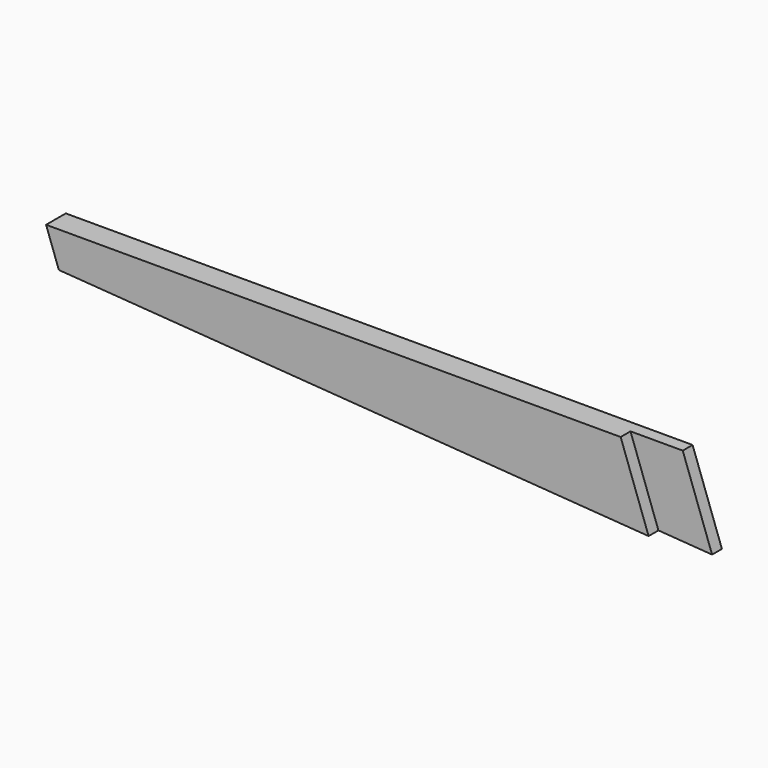
from build123d import *

# Parameters (mm, degrees)
F0_W     = 508
F0_H     = 63.5
F1_DEPTH = 19.05
F3_DEPTH = 50.8
F5_DEPTH = 50.8
F7_DEPTH = 38.1
F9_DEPTH = 38.1


with BuildPart() as f1:
    # F0 (on Front) → F1 (new body)
    with BuildSketch(Plane.XZ):
        with Locations((7.0352284261, 31.75)):
            Rectangle(F0_W, F0_H)
    extrude(amount=F1_DEPTH)

    # F2 (on face) → F3 (cut)
    with BuildSketch(Plane.XZ.offset(19.05)):
        Polygon((-224.2599035735, 0), (-246.9647715739, 63.5), (-246.9647715739, 0), align=None)
    extrude(amount=-F3_DEPTH, mode=Mode.SUBTRACT)

    # F4 (on face) → F5 (cut)
    with BuildSketch(Plane.XZ.offset(19.05)):
        Polygon((261.0352284261, 0), (-237.0874956021, 35.8756586385), (-224.2599035735, 0), align=None)
    extrude(amount=-F5_DEPTH, mode=Mode.SUBTRACT)

    # F6 (on face) → F7 (cut)
    with BuildSketch(Plane.XZ.offset(19.05)):
        Polygon((238.3303604257, 63.5), (261.0352284261, 0), (261.0352284261, 63.5), align=None)
    extrude(amount=-F7_DEPTH, mode=Mode.SUBTRACT)

    # F8 (on face) → F9 (cut)
    with BuildSketch(Plane(origin=(231.445604258, 0, 82.7549904558), x_dir=(0, 1, 0), z_dir=(0.941618337, 0, 0.3366822055))):
        Polygon((-19.05, 40.5242251848), (-19.05, -87.885916413), (-9.525, -87.885916413), (-9.525, 37.3283624649), align=None)
    extrude(amount=-F9_DEPTH, mode=Mode.SUBTRACT)


solid = f1.part
